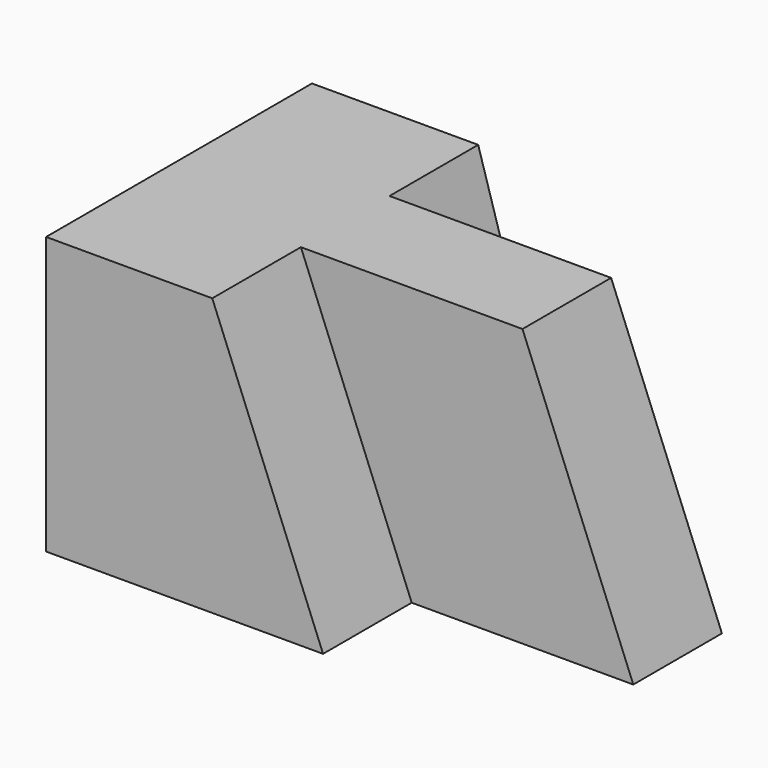
from build123d import *

# Parameters (mm, degrees)
F0_W     = 57.15
F0_H     = 31.75
F1_DEPTH = 38.1
F3_DEPTH = 38.1
F5_DEPTH = 12.7
F7_DEPTH = 12.7


# Not quite as in the source:
# - a length typed as a fraction of an inch, garbled in the dataset ("3 / 203.2 mm" for 3/8 in), is restored


with BuildPart() as f1:
    # F0 (on Front) → F1 (new body)
    with BuildSketch(Plane.XZ):
        with Locations((28.575, 15.875)):
            Rectangle(F0_W, F0_H)
    extrude(amount=F1_DEPTH)

    # F2 (on face) → F3 (cut)
    with BuildSketch(Plane.XZ.offset(38.1)):
        Polygon((44.45, 31.75), (57.15, 0), (57.15, 31.75), align=None)
    extrude(amount=-F3_DEPTH, mode=Mode.SUBTRACT)

    # F4 (on face) → F5 (cut)
    with BuildSketch(Plane(origin=(0, 0, 0), x_dir=(-1, 0, 0), z_dir=(0, 1, 0))):
        Polygon((-44.45, 31.75), (-57.15, 0), (-28.575, 0), (-19.05, 31.75), align=None)
    extrude(amount=-F5_DEPTH, mode=Mode.SUBTRACT)

    # F6 (on face) → F7 (cut)
    with BuildSketch(Plane.XZ.offset(38.1)):
        Polygon((31.75, 0), (57.15, 0), (44.45, 31.75), (19.05, 31.75), align=None)
    extrude(amount=-F7_DEPTH, mode=Mode.SUBTRACT)


solid = f1.part
